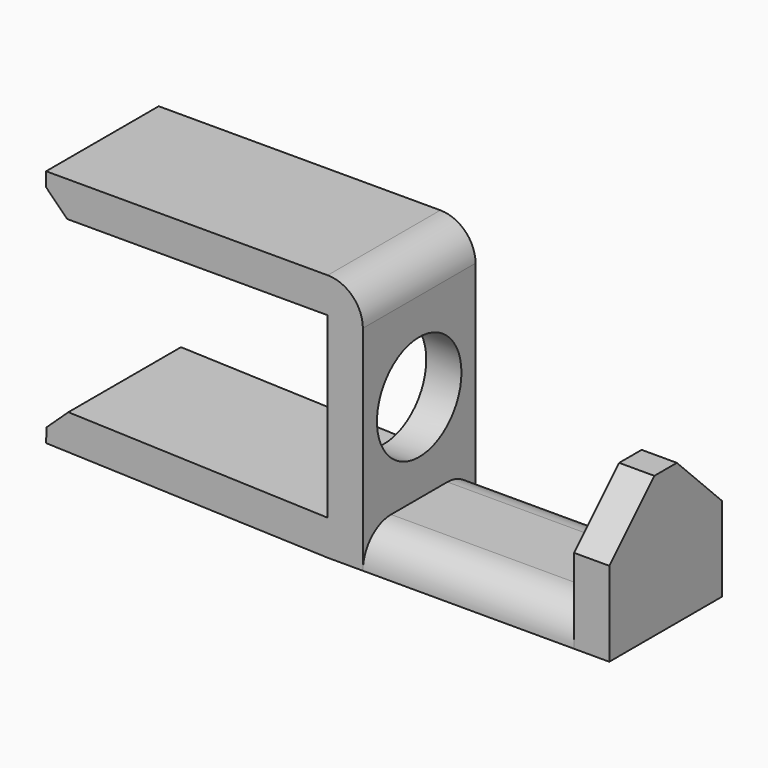
from build123d import *

# Parameters (mm, degrees)
F0_W           = 40
F0_H           = 5
F0_W_2         = 30
F1_DEPTH       = 20
F2_R           = 4.99999
F3_SIZE        = 3
F5_D           = 15
F5_DEPTH       = 20
F5_CBORE_D     = 15
F5_CBORE_DEPTH = 5
F5_TIP         = 4.5064546427
F6_SIZE        = 8


# Not quite as in the source:
# - a fillet or chamfer is up to 0.001 mm smaller than in the source, because OpenCascade refuses the exact size


with BuildPart() as f1:
    # F0 (on Front) → F1 (new body)
    with BuildSketch(Plane.XZ):
        with Locations((-20, 50.4448633795)):
            Rectangle(F0_W, F0_H)
        Polygon((5, 52.9448633795), (0, 52.9448633795), (0, 47.9448633795), (0, 22.6232533795), (0, 17.6205022253), (5, 17.6205022253), (5, 22.6205022253), align=None)
        Polygon((0, 17.6205022253), (0, 22.6232533795), (-39.8342023775, 23.9448633795), (-40, 18.9476130207), align=None)
        with Locations((20, 20.1205022253)):
            Rectangle(F0_W_2, F0_H)
        Polygon((35, 37.6205022253), (35, 22.6205022253), (35, 17.6205022253), (40, 17.6205022253), (40, 37.6205022253), align=None)
    extrude(amount=F1_DEPTH)

    # F2 (radius 5 in the source; OpenCascade refuses exactly that, so slightly less here)
    f2_edges = [f1.edges().sort_by_distance(p)[0] for p in [
        (20, -20, 22.620502),
        (20, 0, 22.620502),
        (5, -10, 52.944863),
    ]]
    fillet(f2_edges, radius=F2_R)

    # F3
    f3_edges = [f1.edges().sort_by_distance(p)[0] for p in [
        (-40, -10, 47.944863),
        (-39.834202, -10, 23.944863),
    ]]
    chamfer(f3_edges, length=F3_SIZE)

    # F5
    with Locations(Plane(origin=(0, 0, 0), x_dir=(0, -1, 0), z_dir=(-1, 0, 0))):
        with Locations((10, 35.2840583795)):
            CounterBoreHole(F5_D / 2, F5_CBORE_D / 2, F5_CBORE_DEPTH, depth=F5_DEPTH)
            with Locations((0, 0, -(F5_DEPTH + F5_TIP / 2))):  # 118° drill point
                Cone(0, F5_D / 2, F5_TIP, mode=Mode.SUBTRACT)

    # F6
    f6_edges = [f1.edges().sort_by_distance(p)[0] for p in [
        (37.5, 0, 37.620502),
        (37.5, -20, 37.620502),
    ]]
    chamfer(f6_edges, length=F6_SIZE)


solid = f1.part
